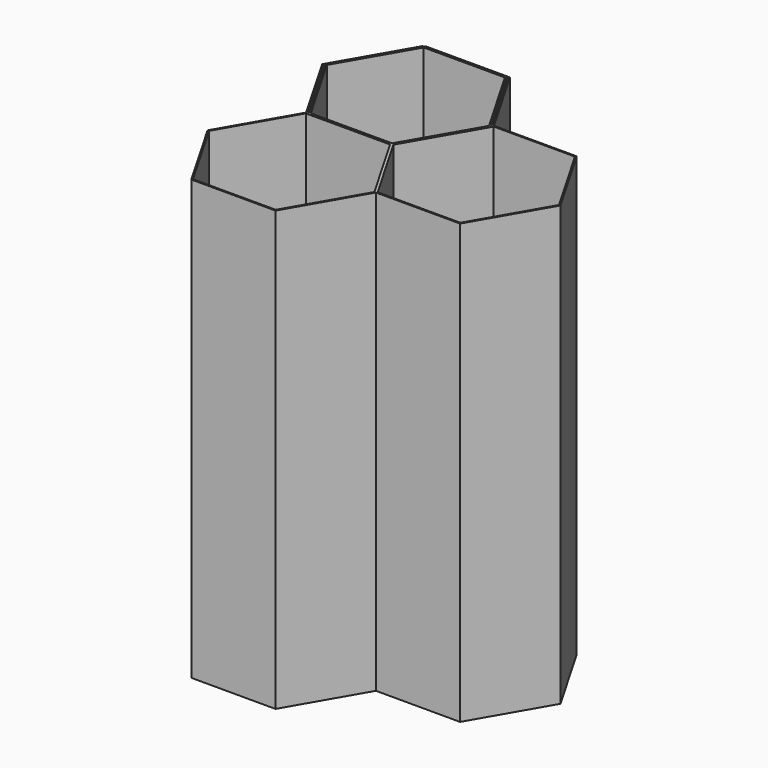
from build123d import *

# Parameters (mm, degrees)
F1_DEPTH = 170
F2_T     = -0.5


# Not quite as in the source:
# - a feature names something its author has since deleted; it is built from what else it names


with BuildPart() as f1:
    # F0 (on Top) → F1 (new body)
    with BuildSketch(Plane.XY):
        Polygon((16.3101451046, 28.25), (-16.3101451046, 28.25), (-32.6202902092, 0), (-16.3101451046, -28.25), (16.3101451046, -28.25), (32.6202902092, 0), align=None)
    extrude(amount=F1_DEPTH)

    # F2
    f2_openings = [f1.faces().sort_by_distance(p)[0] for p in [
        (0, 0, 170),
    ]]
    offset(amount=F2_T, openings=f2_openings)

    # F3: F1 across face


with BuildPart() as f1_1:
    add(f1.part)
    add(f1.part.mirror(Plane(origin=(-24.032204955, 13.875, 85.25), x_dir=(0.5, 0.8660254038, 0), z_dir=(0.8660254038, -0.5, 0))))

    # F4: F1 across face


with BuildPart() as f1_2:
    add(f1_1.part)
    add(f1_1.part.mirror(Plane(origin=(-24.3208800896, -14.375, 85), x_dir=(0.5, -0.8660254038, 0), z_dir=(-0.8660254038, -0.5, 0))))


solid = f1_2.part
